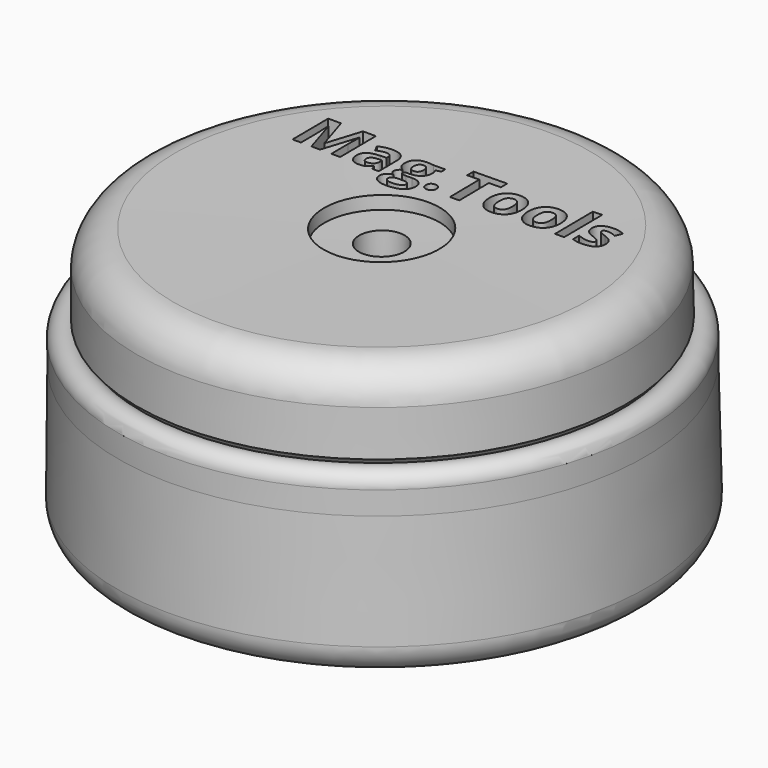
from build123d import *

# Parameters (mm, degrees)
F4_TEXT_SIZE = 3.4301431798
F5_DEPTH     = 15


# Not quite as in the source:
# - Text() gives the source's letters only with a copy of the font that has no kerning and outlines rounded to 1/6400 em; it was checked with that copy


with BuildPart() as f2:
    # F0 (on Front) → F2 (revolve)
    with BuildSketch(Plane.XZ):
        with BuildLine():
            Line((-1.3487565264, 7.9544333927), (-3.1521232403, 7.9434764208))
            Line((-3.1521232403, 7.9434764208), (-3.1521232403, 1.5934764208))
            Line((-3.1521232403, 1.5934764208), (-12.9311232403, 1.5993540598))
            Line((-12.9311232403, 1.5993540598), (-12.9072057985, 6.4858209717))
            Line((-12.9072057985, 6.4858209717), (-12.9072057985, 9.1265536233))
            ThreePointArc((-12.9072057985, 9.1265536233), (-13.709005966, 9.9213191128), (-14.4966750605, 9.1125465308))
            Line((-14.4966750605, 9.1125465308), (-14.4742932171, 7.8427437693))
            Line((-14.4742932171, 7.8427437693), (-14.5186232403, 1.5922685852))
            ThreePointArc((-14.5186232403, 1.5922685852), (-14.0507352368, 0.4747337572), (-12.9311232403, 0.0118382476))
            Line((-12.9311232403, 0.0118382476), (0, 0))
            Line((0, 0), (-0.0152662604, 1.5993382476))
            Line((-0.0152662604, 1.5993382476), (-1.3487565264, 1.6044333927))
            Line((-1.3487565264, 1.6044333927), (-1.3487565264, 7.9544333927))
        make_face()
    revolve(axis=Axis((-0.0076331302, 0, 0.7996691238), (-0.0095449258, 0, 0.9999544462)))


with BuildPart() as f3:
    # F1 (on Front) → F3 (revolve)
    with BuildSketch(Plane.XZ):
        with BuildLine():
            Line((-12.6935122535, 8.3888908848), (-9.5351571217, 8.3593046293))
            Line((-9.5351571217, 8.3593046293), (-9.5351571217, 11.4028118551))
            Line((-9.5351571217, 11.4028118551), (-1.372677274, 11.4028118551))
            Line((-1.372677274, 11.4028118551), (-1.372677274, 13.7276081368))
            Line((-1.372677274, 13.7276081368), (-3.2747837249, 13.7276081368))
            Line((-3.2747837249, 13.7276081368), (-3.2982663251, 14.4350982725))
            Line((-3.2982663251, 14.4350982725), (-11.470278725, 14.4478557631))
            ThreePointArc((-11.470278725, 14.4478557631), (-12.846220754, 13.8988644377), (-13.466315344, 12.5534683466))
            Line((-13.466315344, 12.5534683466), (-13.466315344, 10.0622076932))
            ThreePointArc((-13.466315344, 10.0622076932), (-12.8947796338, 9.6808417755), (-12.6935122535, 9.0238908848))
            Line((-12.6935122535, 9.0238908848), (-12.6935122535, 8.3888908848))
        make_face()
    revolve(axis=Axis((-0.0076331302, 0, 0.7996691238), (-0.0095449258, 0, 0.9999544462)))


with BuildPart() as f5_tool:
    # F4 (on Top) → F5 (new body)
    with BuildSketch(Plane.XY):
        with Locations((-8.6183380336, 4.0923506021)):
            Text('Mag.Tools', F4_TEXT_SIZE, font='Open Sans', font_style=FontStyle.BOLD, text_align=(TextAlign.LEFT, TextAlign.BOTTOM))
    extrude(amount=F5_DEPTH)


with BuildPart() as f2_1:
    add(f2.part)

    # F5: cut by f5_tool
    add(f5_tool.part, mode=Mode.SUBTRACT)


with BuildPart() as f3_1:
    add(f3.part)

    # F5: cut by f5_tool
    add(f5_tool.part, mode=Mode.SUBTRACT)


solid = Compound([f2_1.part, f3_1.part])
